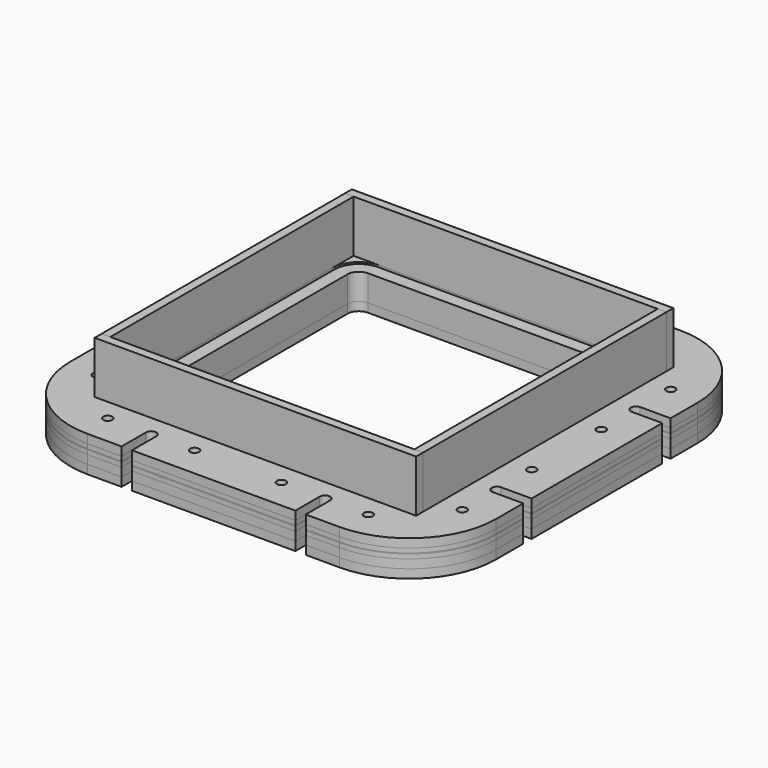
from build123d import *

# Parameters (mm, degrees)
F1_DEPTH  = 5
F3_DEPTH  = 2.5
F5_DEPTH  = 30
F7_DEPTH  = 30
F8_DEPTH  = 0.5
F9_DEPTH  = 2.5
F10_DEPTH = 5
F12_DEPTH = 15
F13_DEPTH = 5
F15_DEPTH = 25
F16_R     = 2.6
F17_DEPTH = 20.501


# Not quite as in the source:
# - a feature names something its author has since deleted; it is built from what else it names


with BuildPart() as f1:
    # F0 (on Top) → F1 (new body)
    with BuildSketch(Plane.XY):
        with BuildLine():
            Line((-72.5, -122.5), (72.5, -122.5))
            ThreePointArc((72.5, -122.5), (107.8553390593, -107.8553390593), (122.5, -72.5))
            Line((122.5, -72.5), (122.5, 72.5))
            ThreePointArc((122.5, 72.5), (107.8553390593, 107.8553390593), (72.5, 122.5))
            Line((72.5, 122.5), (-72.5, 122.5))
            ThreePointArc((-72.5, 122.5), (-107.8553390593, 107.8553390593), (-122.5, 72.5))
            Line((-122.5, 72.5), (-122.5, -72.5))
            ThreePointArc((-122.5, -72.5), (-107.8553390593, -107.8553390593), (-72.5, -122.5))
        make_face()
        with BuildLine():
            ThreePointArc((87.5, -72.5), (83.1066017178, -83.1066017178), (72.5, -87.5))
            Line((72.5, -87.5), (-72.5, -87.5))
            ThreePointArc((-72.5, -87.5), (-83.1066017178, -83.1066017178), (-87.5, -72.5))
            Line((-87.5, -72.5), (-87.5, 72.5))
            ThreePointArc((-87.5, 72.5), (-83.1066017178, 83.1066017178), (-72.5, 87.5))
            Line((-72.5, 87.5), (72.5, 87.5))
            ThreePointArc((72.5, 87.5), (83.1066017178, 83.1066017178), (87.5, 72.5))
            Line((87.5, 72.5), (87.5, -72.5))
        make_face(mode=Mode.SUBTRACT)
    extrude(amount=F1_DEPTH)


with BuildPart() as f3:
    # F2 (on face) → F3 (new body)
    with BuildSketch(Plane(origin=(0, 0, 0), x_dir=(1, 0, 0), z_dir=(0, 0, -1))):
        with BuildLine():
            ThreePointArc((-72.5, 122.5), (-107.8553390593, 107.8553390593), (-122.5, 72.5))
            Line((-122.5, 72.5), (-122.5, -72.5))
            ThreePointArc((-122.5, -72.5), (-107.8553390593, -107.8553390593), (-72.5, -122.5))
            Line((-72.5, -122.5), (72.5, -122.5))
            ThreePointArc((72.5, -122.5), (107.8553390593, -107.8553390593), (122.5, -72.5))
            Line((122.5, -72.5), (122.5, 72.5))
            ThreePointArc((122.5, 72.5), (107.8553390593, 107.8553390593), (72.5, 122.5))
            Line((72.5, 122.5), (-72.5, 122.5))
        make_face()
        with BuildLine():
            Line((-72.5, 87.5), (72.5, 87.5))
            ThreePointArc((72.5, 87.5), (83.1066017178, 83.1066017178), (87.5, 72.5))
            Line((87.5, 72.5), (87.5, -72.5))
            ThreePointArc((87.5, -72.5), (83.1066017178, -83.1066017178), (72.5, -87.5))
            Line((72.5, -87.5), (-72.5, -87.5))
            ThreePointArc((-72.5, -87.5), (-83.1066017178, -83.1066017178), (-87.5, -72.5))
            Line((-87.5, -72.5), (-87.5, 72.5))
            ThreePointArc((-87.5, 72.5), (-83.1066017178, 83.1066017178), (-72.5, 87.5))
        make_face(mode=Mode.SUBTRACT)
    extrude(amount=F3_DEPTH)


with BuildPart() as f5:
    # F4 (on face) → F5 (new body)
    with BuildSketch(Plane.XY.offset(5)):
        Polygon((-92.5, 92.5), (-92.5, 87.5), (-87.5, 87.5), (-72.5, 87.5), (72.5, 87.5), (87.5, 87.5), (92.5, 87.5), (92.5, 92.5), align=None)
    extrude(amount=F5_DEPTH)


with BuildPart() as f5b:
    # F4 (on face) → F5, piece 2 (new body)
    with BuildSketch(Plane.XY.offset(5)):
        Polygon((-87.5, -87.5), (-92.5, -87.5), (-92.5, -92.5), (92.5, -92.5), (92.5, -87.5), (87.5, -87.5), (72.5, -87.5), (-72.5, -87.5), align=None)
    extrude(amount=F5_DEPTH)


with BuildPart() as f7:
    # F6 (on face) → F7 (new body)
    with BuildSketch(Plane.XY.offset(5)):
        Polygon((-87.5, -72.5), (-87.5, 72.5), (-87.5, 87.5), (-92.5, 87.5), (-92.5, -87.5), (-87.5, -87.5), align=None)
    extrude(amount=F7_DEPTH)


with BuildPart() as f7b:
    # F6 (on face) → F7, piece 2 (new body)
    with BuildSketch(Plane.XY.offset(5)):
        Polygon((92.5, 87.5), (87.5, 87.5), (87.5, 72.5), (87.5, -72.5), (87.5, -87.5), (92.5, -87.5), align=None)
    extrude(amount=F7_DEPTH)


with BuildPart() as f8:
    # F8 (new): a face of the model
    f8_faces = [f3.part.faces().sort_by_distance(p)[0] for p in [
        (-105.4053390593, -105.4053390593, -2.5),
    ]]
    extrude(f8_faces, amount=F8_DEPTH)


with BuildPart() as f9:
    # F9 (new): a face of the model
    f9_faces = [f8.part.faces().sort_by_distance(p)[0] for p in [
        (-105.4053390593, -105.4053390593, -3),
    ]]
    extrude(f9_faces, amount=F9_DEPTH)


with BuildPart() as f10:
    # F10 (new): a face of the model
    f10_faces = [f9.part.faces().sort_by_distance(p)[0] for p in [
        (-105.4053390593, -105.4053390593, -5.5),
    ]]
    extrude(f10_faces, amount=F10_DEPTH)


with BuildPart() as f12:
    # F11 (on face) → F12 (new body)
    with BuildSketch(Plane(origin=(0, 0, -10.5), x_dir=(1, 0, 0), z_dir=(0, 0, -1))):
        with BuildLine():
            ThreePointArc((86.5, 72.5), (82.3994949366, 82.3994949366), (72.5, 86.5))
            Line((72.5, 86.5), (-72.5, 86.5))
            ThreePointArc((-72.5, 86.5), (-82.3994949366, 82.3994949366), (-86.5, 72.5))
            Line((-86.5, 72.5), (-86.5, -72.5))
            ThreePointArc((-86.5, -72.5), (-82.3994949366, -82.3994949366), (-72.5, -86.5))
            Line((-72.5, -86.5), (72.5, -86.5))
            ThreePointArc((72.5, -86.5), (82.3994949366, -82.3994949366), (86.5, -72.5))
            Line((86.5, -72.5), (86.5, 72.5))
        make_face()
        with BuildLine():
            Line((-72.5, 79), (72.5, 79))
            ThreePointArc((72.5, 79), (77.0961940777, 77.0961940777), (79, 72.5))
            Line((79, 72.5), (79, -72.5))
            ThreePointArc((79, -72.5), (77.0961940777, -77.0961940777), (72.5, -79))
            Line((72.5, -79), (-72.5, -79))
            ThreePointArc((-72.5, -79), (-77.0961940777, -77.0961940777), (-79, -72.5))
            Line((-79, -72.5), (-79, 72.5))
            ThreePointArc((-79, 72.5), (-77.0961940777, 77.0961940777), (-72.5, 79))
        make_face(mode=Mode.SUBTRACT)
    extrude(amount=-F12_DEPTH)


with BuildPart() as f13:
    # F11 (on face) → F13 (new body)
    with BuildSketch(Plane(origin=(0, 0, -10.5), x_dir=(1, 0, 0), z_dir=(0, 0, -1))):
        with BuildLine():
            ThreePointArc((122.5, 72.5), (107.8553390593, 107.8553390593), (72.5, 122.5))
            Line((72.5, 122.5), (-72.5, 122.5))
            ThreePointArc((-72.5, 122.5), (-107.8553390593, 107.8553390593), (-122.5, 72.5))
            Line((-122.5, 72.5), (-122.5, -72.5))
            ThreePointArc((-122.5, -72.5), (-107.8553390593, -107.8553390593), (-72.5, -122.5))
            Line((-72.5, -122.5), (72.5, -122.5))
            ThreePointArc((72.5, -122.5), (107.8553390593, -107.8553390593), (122.5, -72.5))
            Line((122.5, -72.5), (122.5, 72.5))
        make_face()
        with BuildLine():
            Line((-72.5, 86.5), (72.5, 86.5))
            ThreePointArc((72.5, 86.5), (82.3994949366, 82.3994949366), (86.5, 72.5))
            Line((86.5, 72.5), (86.5, -72.5))
            ThreePointArc((86.5, -72.5), (82.3994949366, -82.3994949366), (72.5, -86.5))
            Line((72.5, -86.5), (-72.5, -86.5))
            ThreePointArc((-72.5, -86.5), (-82.3994949366, -82.3994949366), (-86.5, -72.5))
            Line((-86.5, -72.5), (-86.5, 72.5))
            ThreePointArc((-86.5, 72.5), (-82.3994949366, 82.3994949366), (-72.5, 86.5))
        make_face(mode=Mode.SUBTRACT)
        with BuildLine():
            ThreePointArc((86.5, 72.5), (82.3994949366, 82.3994949366), (72.5, 86.5))
            Line((72.5, 86.5), (-72.5, 86.5))
            ThreePointArc((-72.5, 86.5), (-82.3994949366, 82.3994949366), (-86.5, 72.5))
            Line((-86.5, 72.5), (-86.5, -72.5))
            ThreePointArc((-86.5, -72.5), (-82.3994949366, -82.3994949366), (-72.5, -86.5))
            Line((-72.5, -86.5), (72.5, -86.5))
            ThreePointArc((72.5, -86.5), (82.3994949366, -82.3994949366), (86.5, -72.5))
            Line((86.5, -72.5), (86.5, 72.5))
        make_face()
        with BuildLine():
            Line((-72.5, 79), (72.5, 79))
            ThreePointArc((72.5, 79), (77.0961940777, 77.0961940777), (79, 72.5))
            Line((79, 72.5), (79, -72.5))
            ThreePointArc((79, -72.5), (77.0961940777, -77.0961940777), (72.5, -79))
            Line((72.5, -79), (-72.5, -79))
            ThreePointArc((-72.5, -79), (-77.0961940777, -77.0961940777), (-79, -72.5))
            Line((-79, -72.5), (-79, 72.5))
            ThreePointArc((-79, 72.5), (-77.0961940777, 77.0961940777), (-72.5, 79))
        make_face(mode=Mode.SUBTRACT)
    extrude(amount=F13_DEPTH)


with BuildPart() as f15_tool:
    # F14 (on face) → F15 (new body)
    with BuildSketch(Plane(origin=(0, 0, -15.5), x_dir=(1, 0, 0), z_dir=(0, 0, -1))):
        with BuildLine():
            Line((53, 122.5), (47, 122.5))
            Line((47, 122.5), (47, 105))
            ThreePointArc((47, 105), (50, 102), (53, 105))
            Line((53, 105), (53, 122.5))
        make_face()
        Polygon((47, 134.1084390879), (47, 122.5), (53, 122.5), (53, 135.0907385349), align=None)
        Polygon((-53, 134.8942816257), (-53, 122.5), (-47, 122.5), (-47, 133.7155252695), align=None)
        with BuildLine():
            Line((-53, 122.5), (-53, 105))
            ThreePointArc((-53, 105), (-50, 102), (-47, 105))
            Line((-47, 105), (-47, 122.5))
            Line((-47, 122.5), (-53, 122.5))
        make_face()
        with BuildLine():
            Line((-105, 53), (-122.5, 53))
            Line((-122.5, 53), (-122.5, 47))
            Line((-122.5, 47), (-105, 47))
            ThreePointArc((-105, 47), (-102, 50), (-105, 53))
        make_face()
        with BuildLine():
            Line((-105, -47), (-122.5, -47))
            Line((-122.5, -47), (-122.5, -53))
            Line((-122.5, -53), (-105, -53))
            ThreePointArc((-105, -53), (-102, -50), (-105, -47))
        make_face()
        with BuildLine():
            Line((-53, -105), (-53, -122.5))
            Line((-53, -122.5), (-47, -122.5))
            Line((-47, -122.5), (-47, -105))
            ThreePointArc((-47, -105), (-50, -102), (-53, -105))
        make_face()
        with BuildLine():
            Line((47, -105), (47, -122.5))
            Line((47, -122.5), (53, -122.5))
            Line((53, -122.5), (53, -105))
            ThreePointArc((53, -105), (50, -102), (47, -105))
        make_face()
        with BuildLine():
            Line((122.5, -53), (122.5, -47))
            Line((122.5, -47), (105, -47))
            ThreePointArc((105, -47), (102, -50), (105, -53))
            Line((105, -53), (122.5, -53))
        make_face()
        with BuildLine():
            Line((122.5, 47), (122.5, 53))
            Line((122.5, 53), (105, 53))
            ThreePointArc((105, 53), (102, 50), (105, 47))
            Line((105, 47), (122.5, 47))
        make_face()
    extrude(amount=-F15_DEPTH)


with BuildPart() as f1_1:
    add(f1.part)

    # F15: cut by f15_tool
    add(f15_tool.part, mode=Mode.SUBTRACT)


with BuildPart() as f3_1:
    add(f3.part)

    # F15: cut by f15_tool
    add(f15_tool.part, mode=Mode.SUBTRACT)


with BuildPart() as f8_1:
    add(f8.part)

    # F15: cut by f15_tool
    add(f15_tool.part, mode=Mode.SUBTRACT)


with BuildPart() as f9_1:
    add(f9.part)

    # F15: cut by f15_tool
    add(f15_tool.part, mode=Mode.SUBTRACT)


with BuildPart() as f10_1:
    add(f10.part)

    # F15: cut by f15_tool
    add(f15_tool.part, mode=Mode.SUBTRACT)


with BuildPart() as f13_1:
    add(f13.part)

    # F15: cut by f15_tool
    add(f15_tool.part, mode=Mode.SUBTRACT)


with BuildPart() as f17_tool:
    # F16 (on face) → F17 (new body, through all)
    with BuildSketch(Plane.XY.offset(5)):
        with Locations((-105, 25)):
            Circle(F16_R)
        with Locations((-105, 75)):
            Circle(F16_R)
        with Locations((-105, -75)):
            Circle(F16_R)
        with Locations((-105, -25)):
            Circle(F16_R)
        with Locations((105, 75)):
            Circle(F16_R)
        with Locations((105, 25)):
            Circle(F16_R)
        with Locations((105, -25)):
            Circle(F16_R)
        with Locations((105, -75)):
            Circle(F16_R)
        with Locations((-25, -105)):
            Circle(F16_R)
        with Locations((25, -105)):
            Circle(F16_R)
        with Locations((75, -105)):
            Circle(F16_R)
        with Locations((-75, -105)):
            Circle(F16_R)
        with Locations((-75, 105)):
            Circle(F16_R)
        with Locations((-25, 105)):
            Circle(F16_R)
        with Locations((25, 105)):
            Circle(F16_R)
        with Locations((75, 105)):
            Circle(F16_R)
    extrude(amount=-F17_DEPTH)


with BuildPart() as f1_2:
    add(f1_1.part)

    # F17: cut by f17_tool
    add(f17_tool.part, mode=Mode.SUBTRACT)


with BuildPart() as f3_2:
    add(f3_1.part)

    # F17: cut by f17_tool
    add(f17_tool.part, mode=Mode.SUBTRACT)


with BuildPart() as f8_2:
    add(f8_1.part)

    # F17: cut by f17_tool
    add(f17_tool.part, mode=Mode.SUBTRACT)


with BuildPart() as f9_2:
    add(f9_1.part)

    # F17: cut by f17_tool
    add(f17_tool.part, mode=Mode.SUBTRACT)


with BuildPart() as f10_2:
    add(f10_1.part)

    # F17: cut by f17_tool
    add(f17_tool.part, mode=Mode.SUBTRACT)


solid = Compound([f5.part, f5b.part, f7.part, f7b.part, f12.part, f13_1.part, f1_2.part, f3_2.part, f8_2.part, f9_2.part, f10_2.part])
